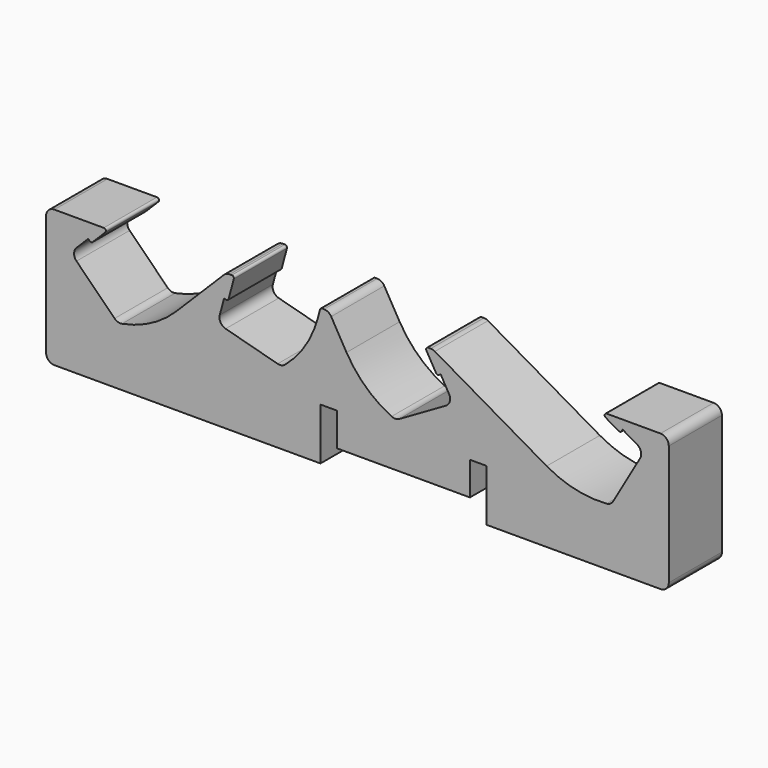
from build123d import *

# Parameters (mm, degrees)
F2_DEPTH = 4
F3_R     = 1
F4_R     = 0.25


# Not quite as in the source:
# - a feature names something its author has since deleted; it is built from what else it names


with BuildPart() as f2:
    # F1 (on Front) → F2 (new body, symmetric)
    with BuildSketch(Plane.XZ):
        with BuildLine():
            Line((-37.5, 16.4951905284), (-37.5, 0))
            Line((-37.5, 0), (-4.4515441619, 0))
            Line((-4.4515441619, 0), (-4.4515441619, 6.25))
            Line((-4.4515441619, 6.25), (-2.4515441619, 6.25))
            Line((-2.4515441619, 6.25), (-2.4515441619, 2.25))
            Line((-2.4515441619, 2.25), (13.5484558381, 2.25))
            Line((13.5484558381, 2.25), (13.5484558381, 6.25))
            Line((13.5484558381, 6.25), (15.5484558381, 6.25))
            Line((15.5484558381, 6.25), (15.5484558381, 0))
            Line((15.5484558381, 0), (37.5, 0))
            Line((37.5, 0), (37.5, 16.4951905284))
            Line((37.5, 16.4951905284), (29.0959722333, 16.4951905284))
            Line((29.0959722333, 16.4951905284), (31.6940484447, 14.9951905284))
            Line((31.6940484447, 14.9951905284), (31.9440484447, 15.4282032303))
            Line((31.9440484447, 15.4282032303), (34.542124656, 13.9282032303))
            Line((34.542124656, 13.9282032303), (30.542124656, 7))
            ThreePointArc((30.542124656, 7), (26.5409294992, 7.164032547), (22.7969341276, 8.5849364905))
            Line((22.7969341276, 8.5849364905), (9.0959722333, 16.4951905284))
            Line((9.0959722333, 16.4951905284), (8.0959722333, 16.4951905284))
            Line((8.0959722333, 16.4951905284), (9.5959722333, 13.897114317))
            Line((9.5959722333, 13.897114317), (10.0289849352, 14.147114317))
            Line((10.0289849352, 14.147114317), (11.5289849352, 11.5490381057))
            Line((11.5289849352, 11.5490381057), (4.6007817049, 7.5490381057))
            ThreePointArc((4.6007817049, 7.5490381057), (1.2176613272, 9.6916920368), (-1.3142818045, 12.7942286341))
            Line((-1.3142818045, 12.7942286341), (-3.4510331505, 16.4951905284))
            Line((-3.4510331505, 16.4951905284), (-4.4510331505, 16.4951905284))
            Line((-4.4510331505, 16.4951905284), (-4.756308124, 15.3558888168))
            ThreePointArc((-4.756308124, 15.3558888168), (-6.3989818261, 11.7037534869), (-9.112265528, 8.7584927324))
            Line((-9.112265528, 8.7584927324), (-16.8396721383, 10.8290450932))
            Line((-16.8396721383, 10.8290450932), (-16.063215003, 13.7268225721))
            Line((-16.063215003, 13.7268225721), (-15.5802520899, 13.5974130495))
            Line((-15.5802520899, 13.5974130495), (-14.8037949546, 16.4951905284))
            Line((-14.8037949546, 16.4951905284), (-15.8037949546, 16.4951905284))
            Line((-15.8037949546, 16.4951905284), (-21.8142025947, 10.4847828883))
            ThreePointArc((-21.8142025947, 10.4847828883), (-25.0628674157, 8.1432777656), (-28.8852704065, 6.9492489824))
            Line((-28.8852704065, 6.9492489824), (-34.542124656, 12.6061032319))
            Line((-34.542124656, 12.6061032319), (-32.4208043125, 14.7274235754))
            Line((-32.4208043125, 14.7274235754), (-32.0672509219, 14.3738701848))
            Line((-32.0672509219, 14.3738701848), (-29.9459305783, 16.4951905284))
            Line((-29.9459305783, 16.4951905284), (-37.5, 16.4951905284))
        make_face()
    extrude(amount=F2_DEPTH, both=True)

    # F3
    f3_edges = [f2.edges().sort_by_distance(p)[0] for p in [
        (-37.5, 0, 0),
        (37.5, 0, 0),
        (37.5, 0, 16.495191),
        (9.095972, 0, 16.495191),
        (30.542125, 0, 7),
        (4.600782, 0, 7.549038),
        (34.542125, 0, 13.928203),
        (-9.112266, 0, 8.758493),
        (-28.88527, 0, 6.949249),
        (-3.451033, 0, 16.495191),
        (-1.314282, 0, 12.794229),
        (-15.803795, 0, 16.495191),
        (-37.5, 0, 16.495191),
        (11.528985, 0, 11.549038),
        (-16.839672, 0, 10.829045),
        (-34.542125, 0, 12.606103),
    ]]
    fillet(f3_edges, radius=F3_R)

    # F4
    f4_edges = [f2.edges().sort_by_distance(p)[0] for p in [
        (29.095972, 0, 16.495191),
        (-4.451033, 0, 16.495191),
        (-14.803795, 0, 16.495191),
        (-29.945931, 0, 16.495191),
        (31.694048, 0, 14.995191),
        (-15.580252, 0, 13.597413),
        (-32.067251, 0, 14.37387),
        (9.595972, 0, 13.897114),
        (8.095972, 0, 16.495191),
    ]]
    fillet(f4_edges, radius=F4_R)


solid = f2.part
